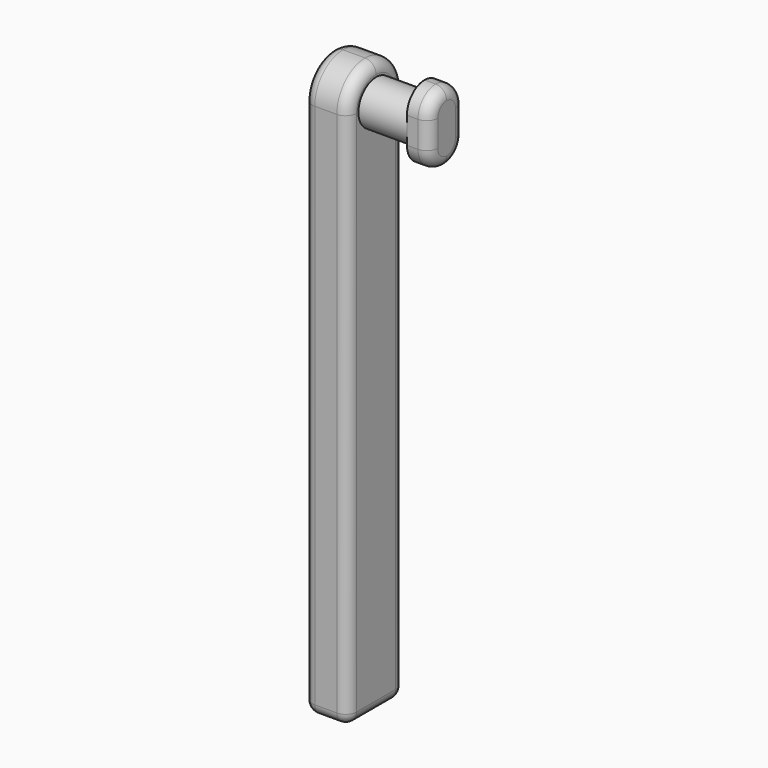
from build123d import *

# Parameters (mm, degrees)
F0_W     = 16
F0_H     = 130
F1_DEPTH = 10
F2_R     = 5
F3_DEPTH = 11
F4_W     = 10
F4_H     = 16
F5_DEPTH = 5
F6_R     = 7.99999
F7_R     = 4.99999
F8_R     = 2.5


# Not quite as in the source:
# - a fillet or chamfer is up to 0.001 mm smaller than in the source, because OpenCascade refuses the exact size


with BuildPart() as f1:
    # F0 (on Right) → F1 (new body)
    with BuildSketch(Plane.YZ):
        with Locations((0, -57)):
            Rectangle(F0_W, F0_H)
    extrude(amount=F1_DEPTH)

    # F2 (on face) → F3 (join)
    with BuildSketch(Plane.YZ.offset(10)):
        Circle(F2_R)
    extrude(amount=F3_DEPTH)

    # F4 (on face) → F5 (join)
    with BuildSketch(Plane.YZ.offset(21)):
        Rectangle(F4_W, F4_H)
    extrude(amount=F5_DEPTH)

    # F6 (radius 8 in the source; OpenCascade refuses exactly that, so slightly less here)
    f6_edges = [f1.edges().sort_by_distance(p)[0] for p in [
        (5, -8, 8),
        (5, 8, 8),
    ]]
    fillet(f6_edges, radius=F6_R)

    # F7 (radius 5 in the source; OpenCascade refuses exactly that, so slightly less here)
    f7_edges = [f1.edges().sort_by_distance(p)[0] for p in [
        (23.5, -5, 8),
        (23.5, 5, 8),
        (23.5, -5, -8),
        (23.5, 5, -8),
    ]]
    fillet(f7_edges, radius=F7_R)

    # F8
    f8_edges = [f1.edges().sort_by_distance(p)[0] for p in [
        (26, 3.535537, 6.535537),
        (10, -5.656857, 5.656857),
        (0, -5.656857, 5.656857),
        (0, 0, -122),
        (5, -8, -122),
        (10, 0, -122),
        (5, 8, -122),
    ]]
    fillet(f8_edges, radius=F8_R)


solid = f1.part
